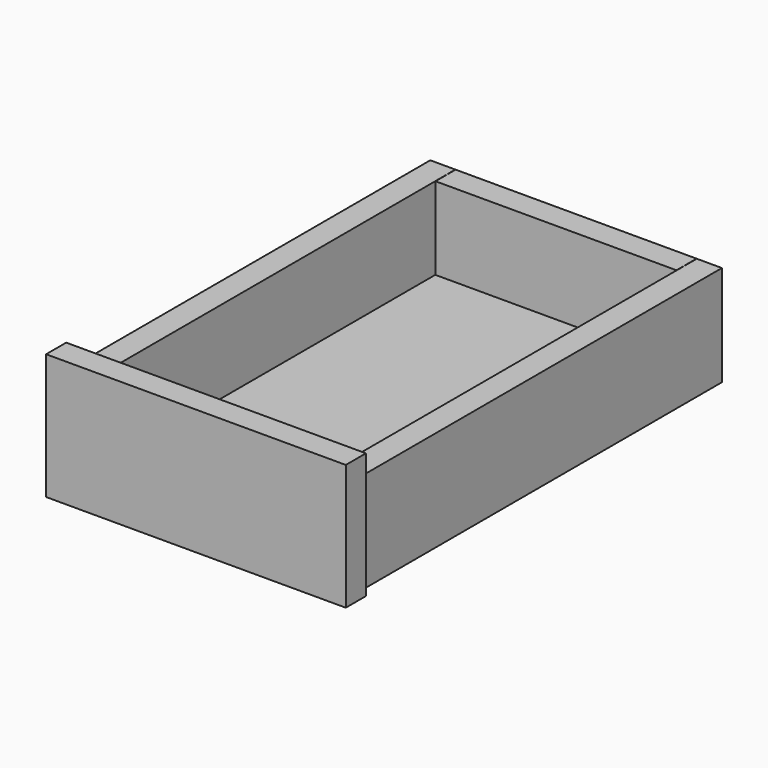
from build123d import *

# Parameters (mm, degrees)
F0_W     = 25
F0_H     = 447.5
F1_DEPTH = 100
F0_W_2   = 239.6
F0_H_2   = 25
F2_W     = 260
F2_H     = 8
F3_DEPTH = 430
F4_W     = 260
F4_H     = 420.9302674979
F5_DEPTH = 8
F6_W     = 298
F6_H     = 125
F7_DEPTH = 25


with BuildPart() as f1:
    # F0 (on Top) → F1 (new body)
    with BuildSketch(Plane.XY):
        with Locations((-284.2940492184, 6.1665456742)):
            Rectangle(F0_W, F0_H)
    extrude(amount=F1_DEPTH)


with BuildPart() as f1b:
    # F0 (on Top) → F1, piece 2 (new body)
    with BuildSketch(Plane.XY):
        with Locations((-19.2940492184, 6.1665456742)):
            Rectangle(F0_W, F0_H)
    extrude(amount=F1_DEPTH)


with BuildPart() as f1c:
    # F0 (on Top) → F1, piece 3 (new body)
    with BuildSketch(Plane.XY):
        with Locations((-151.7940492184, 217.4165456742)):
            Rectangle(F0_W_2, F0_H_2)
    extrude(amount=F1_DEPTH)


with BuildPart() as f1d:
    # F0 (on Top) → F1, piece 4 (new body)
    with BuildSketch(Plane.XY):
        with Locations((-151.7940492184, -205.0834543258)):
            Rectangle(F0_W_2, F0_H_2)
    extrude(amount=F1_DEPTH)


with BuildPart() as f3_tool:
    # F2 (on face) → F3 (new body)
    with BuildSketch(Plane.XZ.offset(217.5834543258)):
        with Locations((-151.7940492184, 14)):
            Rectangle(F2_W, F2_H)
    extrude(amount=-F3_DEPTH)


with BuildPart() as f1_1:
    add(f1.part)

    # F3: cut by f3_tool
    add(f3_tool.part, mode=Mode.SUBTRACT)


with BuildPart() as f1b_1:
    add(f1b.part)

    # F3: cut by f3_tool
    add(f3_tool.part, mode=Mode.SUBTRACT)


with BuildPart() as f1c_1:
    add(f1c.part)

    # F3: cut by f3_tool
    add(f3_tool.part, mode=Mode.SUBTRACT)


with BuildPart() as f5:
    # F4 (on face) → F5 (new body)
    with BuildSketch(Plane.XY.offset(10)):
        with Locations((-151.7940492184, 1.9514119253)):
            Rectangle(F4_W, F4_H)
    extrude(amount=F5_DEPTH)


with BuildPart() as f7:
    # F6 (on face) → F7 (new body)
    with BuildSketch(Plane.XZ.offset(217.5834543258)):
        with Locations((-151.7940492184, 58.5)):
            Rectangle(F6_W, F6_H)
    extrude(amount=F7_DEPTH)


solid = Compound([f1d.part, f1_1.part, f1b_1.part, f1c_1.part, f5.part, f7.part])
